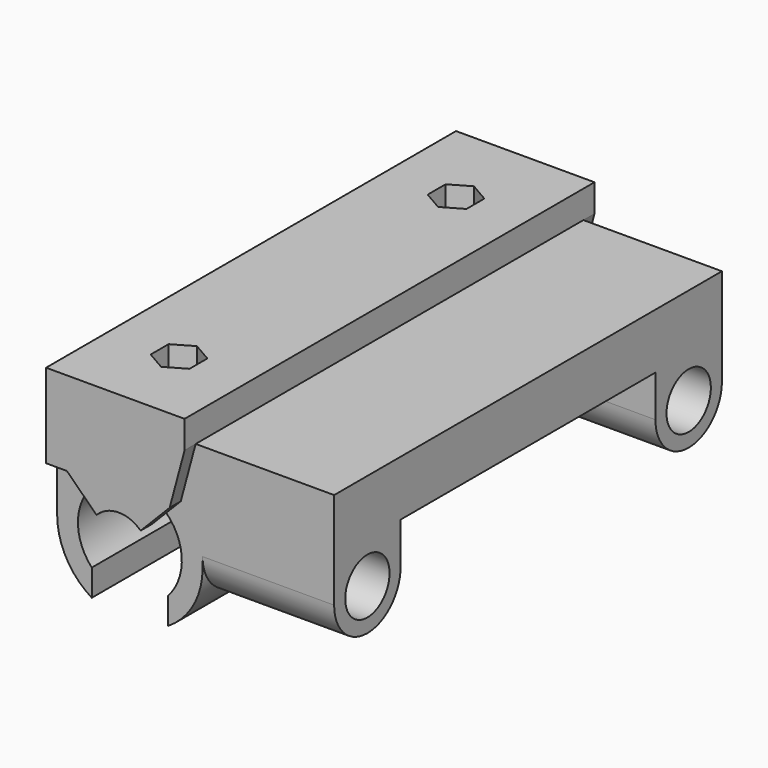
from build123d import *

# Parameters (mm, degrees)
F1_DEPTH  = 70
F3_DEPTH  = 24
F6_DEPTH  = 2
F8_R      = 4
F9_DEPTH  = 19
F11_DEPTH = 3.5


# Not quite as in the source:
# - a pattern or mirror of a feature is missing from the dataset's text; its kind, count and spacing are read off the source's solid


with BuildPart() as f1:
    # F0 (on Front) → F1 (new body)
    with BuildSketch(Plane.XZ):
        Polygon((-20, -12), (20, -12), (20, -4), (0, -4), (0, 0), (-20, 0), (-20, -4), align=None)
    extrude(amount=F1_DEPTH)

    # F2 (on face) → F3 (join)
    with BuildSketch(Plane.XZ.offset(70)):
        with BuildLine():
            ThreePointArc((-15, -24.5990195136), (-16.3735960923, -16.4993872692), (-9.5000000231, -12))
            Line((-9.5000000231, -12), (-20, -12))
            Line((-20, -12), (-20, -19.5))
            ThreePointArc((-20, -19.5), (-18.6651513899, -24.623475383), (-15, -28.44427191))
            Line((-15, -28.44427191), (-15, -24.5990195136))
        make_face()
        with BuildLine():
            ThreePointArc((-9.5000000231, -12), (-2.626403917, -16.499387248), (-4, -24.5990195136))
            Line((-4, -24.5990195136), (-4, -28.44427191))
            ThreePointArc((-4, -28.44427191), (-0.3348486101, -24.623475383), (1, -19.5))
            Line((1, -19.5), (1, -12))
            Line((1, -12), (-9.5000000231, -12))
        make_face()
    f3 = extrude(amount=-F3_DEPTH)

    # F3_copies: F3 across plane
    add(f3.mirror(Plane.ZX.offset(-35)))

    # F5 (on face) → F6 (join)
    with BuildSketch(Plane.XZ.offset(70)):
        with BuildLine():
            Line((-17, -12.1515307717), (-12.7142857143, -16.350656045))
            ThreePointArc((-12.7142857143, -16.350656045), (-9.5459207584, -15.0002343079), (-6.350656045, -16.2857142857))
            Line((-6.350656045, -16.2857142857), (-2.1515307717, -12))
            Line((-2.1515307717, -12), (0, -4))
            Line((0, -4), (0, 0))
            Line((0, 0), (-20, 0))
            Line((-20, 0), (-20, -12.1515307717))
            Line((-20, -12.1515307717), (-17, -12.1515307717))
        make_face()
    f6 = extrude(amount=F6_DEPTH)

    # F6_copies: F6 across plane
    add(f6.mirror(Plane.ZX.offset(-35)))

    # F6_copies1: F6 across plane
    add(f6.mirror(Plane.ZX.offset(-58)))

    # F6_copies2: F6 across plane
    add(f6.mirror(Plane.ZX.offset(-48)))

    # F8 (on face) → F9 (join, through all)
    with BuildSketch(Plane.YZ.offset(20)):
        with BuildLine():
            Line((-70, -12), (-70, -18))
            ThreePointArc((-70, -18), (-64, -24), (-58, -18))
            Line((-58, -18), (-58, -12))
            Line((-58, -12), (-70, -12))
        make_face()
        with Locations((-64, -18)):
            Circle(F8_R, mode=Mode.SUBTRACT)
    f9 = extrude(amount=-F9_DEPTH)

    # F9_copies: F9 across plane
    add(f9.mirror(Plane.ZX.offset(-35)))

    # F10 (on face) → F11 (cut)
    with BuildSketch(Plane.XY):
        Polygon((-7.2, -12.1165807537), (-7.2, -8.8834192463), (-10, -7.2668384925), (-12.8, -8.8834192463), (-12.8, -12.1165807537), (-10, -13.7331615075), align=None)
        Polygon((-7.2, -62.1165807537), (-7.2, -58.8834192463), (-10, -57.2668384925), (-12.8, -58.8834192463), (-12.8, -62.1165807537), (-10, -63.7331615075), align=None)
    extrude(amount=-F11_DEPTH, mode=Mode.SUBTRACT)


solid = f1.part
